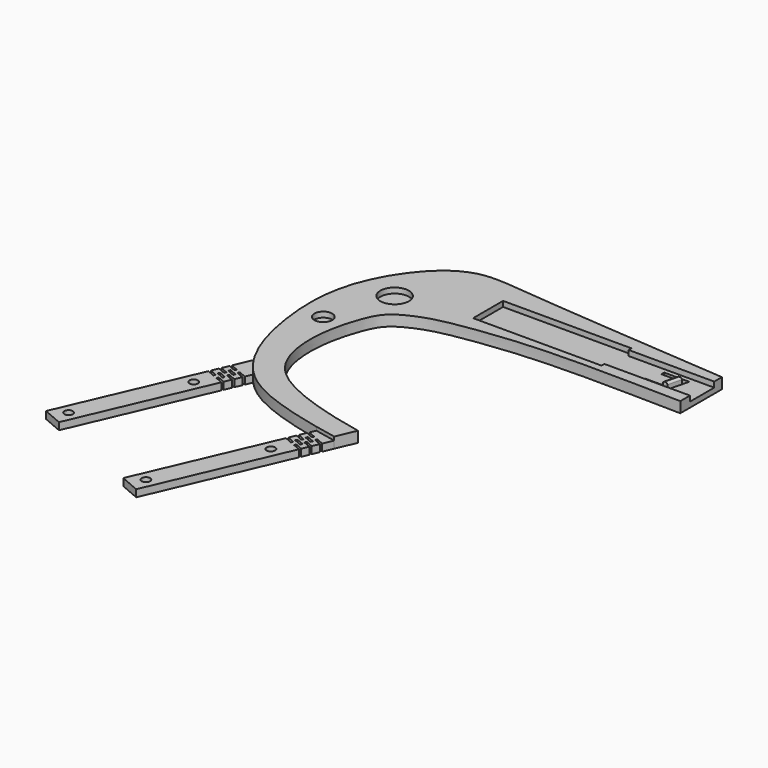
from build123d import *

# Parameters (mm, degrees)
F1_DEPTH = 3
F2_W     = 8.5
F2_H     = 1.5
F3_DEPTH = 60
F0_R     = 1.190625
F4_DEPTH = 2
F6_DEPTH = 1
F7_R     = 0.5
F8_W     = 36
F8_H     = 1
F8_R     = 4
F8_R_2   = 2.5
F9_DEPTH = 1.5


with BuildPart() as f1:
    # F0 (on Top) → F1 (new body)
    with BuildSketch(Plane.XY):
        with BuildLine():
            Line((26.4329920983, -29.1764834751), (28.7654289259, -23.7704801999))
            add(Edge.make_bspline(
                [(28.7654289259, -23.7704801999), (25.4555594803, -23.0757479442), (18.122091552, -21.4647883009), (4.3980129119, -16.8011940655), (-3.8665706509, -10.0291223028), (-6.7654679647, -0.4356418155), (-6.3753072829, 9.6024678508), (-3.6369552871, 18.9389051335), (-0.8623211451, 23.7353358816), (4.7349516236, 26.5836641266), (10.7286597258, 28.5670237026), (24.0928479086, 30.5210675073), (41.0858980443, 31.9179492856), (62.923501486, 31.4689886818), (75.1103142806, 31.2531887853)],
                knots=[0, 0, 0, 0, 0.081391067, 0.1753097966, 0.2544212132, 0.3301545218, 0.4090033083, 0.485425653, 0.5423710265, 0.6017281651, 0.6638442011, 0.7520826863, 0.8549178005, 1, 1, 1, 1], degree=3))
            Line((75.1103142806, 31.2531887853), (75.1103142806, 45.8402432411))
            add(Edge.make_bspline(
                [(-11.0765215286, -10.0946031237), (-11.4039789468, -9.5103994177), (-14.0433837385, -4.4726707186), (-17.1777421826, 6.8494336444), (-18.2575205417, 26.8395665887), (-9.0571179008, 43.867485681), (2.1971560219, 52.1508367912), (18.5095094509, 50.0777693112), (52.5280811409, 47.5313397047), (75.1103142806, 45.8402432411)],
                knots=[0.2825074418, 0.2825074418, 0.2825074418, 0.2825074418, 0.2960030581, 0.3968148217, 0.5097204734, 0.6197990481, 0.7086853513, 0.8057956779, 1, 1, 1, 1], degree=3))
            add(Edge.make_bspline(
                [(-7.0005038153, -15.7930626635), (-8.5837156837, -14.0639344868), (-9.927604005, -12.1443410066), (-11.0765215286, -10.0946031237)],
                knots=[0.2351567051, 0.2351567051, 0.2351567051, 0.2351567051, 0.2825074418, 0.2825074418, 0.2825074418, 0.2825074418], degree=3))
            add(Edge.make_bspline(
                [(20.4258410741, -27.9539063604), (17.7622799682, -27.3661660643), (9.5896661153, -25.3679227855), (-0.7420393691, -21.6766195538), (-5.8549862066, -17.0441566035), (-7.0005038153, -15.7930626635)],
                knots=[0.0430431389, 0.0430431389, 0.0430431389, 0.0430431389, 0.0973147298, 0.2008965382, 0.2351567051, 0.2351567051, 0.2351567051, 0.2351567051], degree=3))
            add(Edge.make_bspline(
                [(26.4329920983, -29.1764834751), (24.5588112261, -28.8237411027), (22.5383280813, -28.4200468729), (20.4258410741, -27.9539063604)],
                knots=[0, 0, 0, 0, 0.0430431389, 0.0430431389, 0.0430431389, 0.0430431389], degree=3))
        make_face()
        Polygon((60.6499973609, 37.0491529702), (66.8692209545, 37.0491529702), (67.8295378742, 40.8904206488), (62.1103142806, 40.8904206488), (62.1103142806, 41.8904206488), (69.1103142806, 41.8904206488), (67.6499973609, 36.0491529702), (60.6499973609, 36.0491529702), align=None, mode=Mode.SUBTRACT)
    extrude(amount=F1_DEPTH)

    # F2 (on face) → F3 (cut)
    with BuildSketch(Plane.YZ.offset(75.1103142806)):
        with Locations((38.8902432411, 2.25)):
            Rectangle(F2_W, F2_H)
    extrude(amount=-F3_DEPTH, mode=Mode.SUBTRACT)

    # F0 (on Top) → F4 (join)
    with BuildSketch(Plane.XY):
        with BuildLine():
            add(Edge.make_bspline(
                [(-7.0005038153, -15.7930626635), (-8.5837156837, -14.0639344868), (-9.927604005, -12.1443410066), (-11.0765215286, -10.0946031237)],
                knots=[0.2351567051, 0.2351567051, 0.2351567051, 0.2351567051, 0.2825074418, 0.2825074418, 0.2825074418, 0.2825074418], degree=3))
            Line((-11.0765215286, -10.0946031237), (-13.3332861786, -15.3252172802))
            Line((-13.3332861786, -15.3252172802), (-11.2214622556, -16.2363702412))
            Line((-11.2214622556, -16.2363702412), (-11.4591543324, -16.7872808298))
            Line((-11.4591543324, -16.7872808298), (-13.5709782553, -15.8761278688))
            Line((-13.5709782553, -15.8761278688), (-14.3632851779, -17.7124964975))
            Line((-14.3632851779, -17.7124964975), (-12.251461255, -18.6236494585))
            Line((-12.251461255, -18.6236494585), (-12.4891533317, -19.1745600471))
            Line((-12.4891533317, -19.1745600471), (-14.6009772547, -18.2634070861))
            Line((-14.6009772547, -18.2634070861), (-15.40134555, -20.1184599538))
            Line((-15.40134555, -20.1184599538), (-13.289521627, -21.0296129148))
            Line((-13.289521627, -21.0296129148), (-13.5272137038, -21.5805235034))
            Line((-13.5272137038, -21.5805235034), (-15.6390376268, -20.6693705424))
            Line((-15.6390376268, -20.6693705424), (-31.5867526479, -57.6321721141))
            Line((-31.5867526479, -57.6321721141), (-26.0776467619, -60.0090928819))
            Line((-26.0776467619, -60.0090928819), (-10.1299317407, -23.0462913102))
            Line((-10.1299317407, -23.0462913102), (-12.2417556637, -22.1351383492))
            Line((-12.2417556637, -22.1351383492), (-12.004063587, -21.5842277606))
            Line((-12.004063587, -21.5842277606), (-9.892239664, -22.4953807216))
            Line((-9.892239664, -22.4953807216), (-9.0918713687, -20.6403278539))
            Line((-9.0918713687, -20.6403278539), (-11.2036952917, -19.7291748929))
            Line((-11.2036952917, -19.7291748929), (-10.9660032149, -19.1782643043))
            Line((-10.9660032149, -19.1782643043), (-8.8541792919, -20.0894172653))
            Line((-8.8541792919, -20.0894172653), (-8.0618723693, -18.2530486366))
            Line((-8.0618723693, -18.2530486366), (-10.1736962923, -17.3418956756))
            Line((-10.1736962923, -17.3418956756), (-9.9360042155, -16.790985087))
            Line((-9.9360042155, -16.790985087), (-7.8241802925, -17.702138048))
            Line((-7.8241802925, -17.702138048), (-7.0005038153, -15.7930626635))
        make_face()
        with Locations((-27.2475858597, -55.1478952406)):
            Circle(F0_R, mode=Mode.SUBTRACT)
        with Locations((-14.9668285594, -26.6841814961)):
            Circle(F0_R, mode=Mode.SUBTRACT)
        Polygon((-13.4253971456, -20.2086148371), (-13.1877050688, -19.6577042485), (-11.0758811458, -20.5688572095), (-11.3135732226, -21.1197677981), align=None, mode=Mode.SUBTRACT)
        Polygon((-12.3873367735, -17.8026513809), (-12.1496446967, -17.2517407922), (-10.0378207737, -18.1628937532), (-10.2755128505, -18.7138043418), align=None, mode=Mode.SUBTRACT)
        with BuildLine():
            Line((25.2522991972, -31.9130333422), (26.4329920983, -29.1764834751))
            add(Edge.make_bspline(
                [(26.4329920983, -29.1764834751), (24.5588112261, -28.8237411027), (22.5383280813, -28.4200468729), (20.4258410741, -27.9539063604)],
                knots=[0, 0, 0, 0, 0.0430431389, 0.0430431389, 0.0430431389, 0.0430431389], degree=3))
            Line((20.4258410741, -27.9539063604), (19.7431933111, -29.5361125744))
            Line((19.7431933111, -29.5361125744), (21.8550172341, -30.4472655354))
            Line((21.8550172341, -30.4472655354), (21.6173251573, -30.998176124))
            Line((21.6173251573, -30.998176124), (19.5055012343, -30.087023163))
            Line((19.5055012343, -30.087023163), (18.7131943117, -31.9233917917))
            Line((18.7131943117, -31.9233917917), (20.8250182347, -32.8345447527))
            Line((20.8250182347, -32.8345447527), (20.5873261579, -33.3854553413))
            Line((20.5873261579, -33.3854553413), (18.475502235, -32.4743023803))
            Line((18.475502235, -32.4743023803), (17.6831953124, -34.310671009))
            Line((17.6831953124, -34.310671009), (19.7950192353, -35.22182397))
            Line((19.7950192353, -35.22182397), (19.5573271586, -35.7727345586))
            Line((19.5573271586, -35.7727345586), (17.4455032356, -34.8615815976))
            Line((17.4455032356, -34.8615815976), (1.4678826683, -71.8936967209))
            Line((1.4678826683, -71.8936967209), (6.9769885544, -74.2706174887))
            Line((6.9769885544, -74.2706174887), (22.9546091216, -37.2385023654))
            Line((22.9546091216, -37.2385023654), (20.8427851986, -36.3273494044))
            Line((20.8427851986, -36.3273494044), (21.0804772754, -35.7764388158))
            Line((21.0804772754, -35.7764388158), (23.1923011984, -36.6875917768))
            Line((23.1923011984, -36.6875917768), (23.984608121, -34.8512231481))
            Line((23.984608121, -34.8512231481), (21.872784198, -33.9400701871))
            Line((21.872784198, -33.9400701871), (22.1104762748, -33.3891595985))
            Line((22.1104762748, -33.3891595985), (24.2223001978, -34.3003125595))
            Line((24.2223001978, -34.3003125595), (25.0146071204, -32.4639439308))
            Line((25.0146071204, -32.4639439308), (22.9027831974, -31.5527909698))
            Line((22.9027831974, -31.5527909698), (23.1404752742, -31.0018803812))
            Line((23.1404752742, -31.0018803812), (25.2522991972, -31.9130333422))
        make_face()
        with Locations((5.8070494566, -69.4094198474)):
            Circle(F0_R, mode=Mode.SUBTRACT)
        with Locations((18.0878067568, -40.9457061029)):
            Circle(F0_R, mode=Mode.SUBTRACT)
        Polygon((19.8968357936, -33.8499153038), (22.0086597166, -34.7610682647), (21.7709676398, -35.3119788533), (19.6591437168, -34.4008258924), align=None, mode=Mode.SUBTRACT)
        Polygon((20.6606983625, -32.0012742707), (20.8983904393, -31.4503636821), (23.0102143623, -32.3615166431), (22.7725222855, -32.9124272317), align=None, mode=Mode.SUBTRACT)
    extrude(amount=F4_DEPTH)

    # F5 (on face) → F6 (join)
    with BuildSketch(Plane.XY.offset(1.5)):
        Polygon((66.572796964, 40.8904206488), (65.6124800444, 37.0491529702), (66.8692209545, 37.0491529702), (67.8295378742, 40.8904206488), align=None)
    extrude(amount=F6_DEPTH)

    # F7
    f7_edges = [f1.edges().sort_by_distance(p)[0] for p in [
        (67.349379, 38.969787, 2.5),
        (66.092639, 38.969787, 2.5),
    ]]
    fillet(f7_edges, radius=F7_R)

    # F8 (on face) → F9 (cut)
    with BuildSketch(Plane.XY.offset(3)):
        with Locations((33.1103142806, 34.1402432411)):
            Rectangle(F8_W, F8_H)
        with Locations((33.1103142806, 43.6402432411)):
            Rectangle(F8_W, F8_H)
        with Locations((-4.8896857194, 31.1402432411)):
            Circle(F8_R)
        with Locations((-10.8896857194, 13.6402432411)):
            Circle(F8_R_2)
    extrude(amount=-F9_DEPTH, mode=Mode.SUBTRACT)


solid = f1.part
